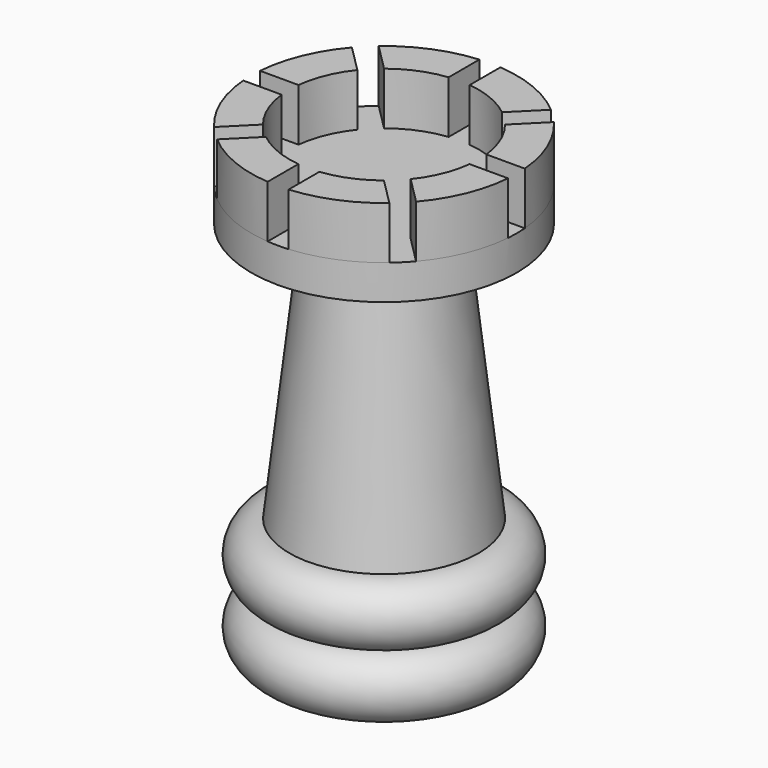
from build123d import *

# Parameters (mm, degrees)
F3_DEPTH = 5


# Not quite as in the source:
# - after a boolean that leaves OpenCascade's solid faulty, fix() repairs it


with BuildPart() as f1:
    # F0 (on Front) → F1 (revolve)
    with BuildSketch(Plane.XZ):
        with BuildLine():
            Line((0, 40), (0, 0))
            Line((0, 0), (9, 0))
            ThreePointArc((9, 0), (12, 3), (9, 6))
            ThreePointArc((9, 6), (12, 9), (9, 12))
            Line((9, 12), (6.4358137697, 34.5418713987))
            Line((6.4358137697, 34.5418713987), (12.6394796214, 36.6926416755))
            Line((12.6394796214, 36.6926416755), (12.6394796214, 40))
            Line((12.6394796214, 40), (0, 40))
        make_face()
    revolve(axis=Axis((0, 0, 20), (0, 0, -1)))

    # F2 (on face) → F3 (join)
    with BuildSketch(Plane.XY.offset(40)):
        with BuildLine():
            ThreePointArc((-8.94427191, 1), (-8.3149157926, 3.4441508913), (-7.0316621015, 5.6174485392))
            Line((-7.0316621015, 5.6174485392), (-9.6165524738, 8.2023389114))
            ThreePointArc((-9.6165524738, 8.2023389114), (-11.6773565238, 4.8369194448), (-12.5998589317, 1))
            Line((-12.5998589317, 1), (-8.94427191, 1))
        make_face()
        with BuildLine():
            ThreePointArc((-1, 12.5998589317), (-4.8369194448, 11.6773565238), (-8.2023389114, 9.6165524738))
            Line((-8.2023389114, 9.6165524738), (-5.6174485392, 7.0316621015))
            ThreePointArc((-5.6174485392, 7.0316621015), (-3.4441508913, 8.3149157926), (-1, 8.94427191))
            Line((-1, 8.94427191), (-1, 12.5998589317))
        make_face()
        with BuildLine():
            ThreePointArc((8.2023389114, 9.6165524738), (4.8369194448, 11.6773565238), (1, 12.5998589317))
            Line((1, 12.5998589317), (1, 8.94427191))
            ThreePointArc((1, 8.94427191), (3.4441508913, 8.3149157926), (5.6174485392, 7.0316621015))
            Line((5.6174485392, 7.0316621015), (8.2023389114, 9.6165524738))
        make_face()
        with BuildLine():
            ThreePointArc((12.5998589317, 1), (11.6773565238, 4.8369194448), (9.6165524738, 8.2023389114))
            Line((9.6165524738, 8.2023389114), (7.0316621015, 5.6174485392))
            ThreePointArc((7.0316621015, 5.6174485392), (8.3149157926, 3.4441508913), (8.94427191, 1))
            Line((8.94427191, 1), (12.5998589317, 1))
        make_face()
        with BuildLine():
            Line((7.0316621015, -5.6174485392), (9.6165524738, -8.2023389114))
            ThreePointArc((9.6165524738, -8.2023389114), (11.6773565238, -4.8369194448), (12.5998589317, -1))
            Line((12.5998589317, -1), (8.94427191, -1))
            ThreePointArc((8.94427191, -1), (8.3149157926, -3.4441508913), (7.0316621015, -5.6174485392))
        make_face()
        with BuildLine():
            Line((1, -8.94427191), (1, -12.5998589317))
            ThreePointArc((1, -12.5998589317), (4.8369194448, -11.6773565238), (8.2023389114, -9.6165524738))
            Line((8.2023389114, -9.6165524738), (5.6174485392, -7.0316621015))
            ThreePointArc((5.6174485392, -7.0316621015), (3.4441508913, -8.3149157926), (1, -8.94427191))
        make_face()
        with BuildLine():
            Line((-5.6174485392, -7.0316621015), (-8.2023389114, -9.6165524738))
            ThreePointArc((-8.2023389114, -9.6165524738), (-4.8369194448, -11.6773565238), (-1, -12.5998589317))
            Line((-1, -12.5998589317), (-1, -8.94427191))
            ThreePointArc((-1, -8.94427191), (-3.4441508913, -8.3149157926), (-5.6174485392, -7.0316621015))
        make_face()
        with BuildLine():
            Line((-8.94427191, -1), (-12.5998589317, -1))
            ThreePointArc((-12.5998589317, -1), (-11.6773565238, -4.8369194448), (-9.6165524738, -8.2023389114))
            Line((-9.6165524738, -8.2023389114), (-7.0316621015, -5.6174485392))
            ThreePointArc((-7.0316621015, -5.6174485392), (-8.3149157926, -3.4441508913), (-8.94427191, -1))
        make_face()
    extrude(amount=F3_DEPTH)

    add(f1.part.fix(), mode=Mode.REPLACE)


solid = f1.part
